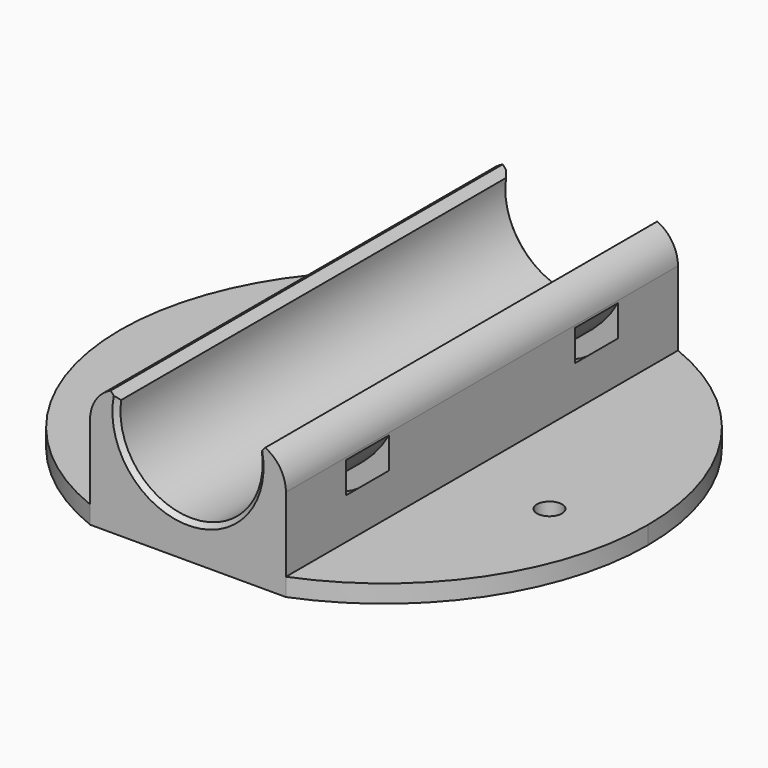
from build123d import *

# Parameters (mm, degrees)
F0_W          = 21.9
F0_H          = 54.784943187
F2_DEPTH      = 13.95
F0_R          = 1.4
F3_DEPTH      = 2
F1_R          = 7.95
F4_DEPTH      = 27.3934715935
F4_DEPTH_BACK = 27.3934715935
F7_R          = 14.5
F7_R_2        = 12.5
F8_R          = 14.5
F8_R_2        = 12.5
F9_DEPTH      = 3
F10_T1_DEPTH  = 59.6298977105
F11_T1_DEPTH  = 72.9200798033
F12_SIZE      = 0.5


# Not quite as in the source:
# - a fillet or chamfer that OpenCascade refuses, or shapes differently, is made with other operations: its cross-section is extruded or revolved along the edge and cut away or added


with BuildPart() as f2:
    # F0 (on Top) → F2 (new body)
    with BuildSketch(Plane.XY):
        Rectangle(F0_W, F0_H)
    extrude(amount=F2_DEPTH)

    # F0 (on Top) → F3 (join)
    with BuildSketch(Plane.XY):
        with BuildLine():
            ThreePointArc((10.95, -27.3924715935), (24.4261642507, -16.5412363504), (29.5, 0))
            ThreePointArc((29.5, 0), (24.4261642507, 16.5412363504), (10.95, 27.3924715935))
            Line((10.95, 27.3924715935), (10.95, -27.3924715935))
        make_face()
        with Locations((20.9, -3)):
            Circle(F0_R, mode=Mode.SUBTRACT)
        with BuildLine():
            Line((-10.95, -27.3924715935), (-10.95, 27.3924715935))
            ThreePointArc((-10.95, 27.3924715935), (-29.5, 0), (-10.95, -27.3924715935))
        make_face()
        with Locations((-20.9, -3)):
            Circle(F0_R, mode=Mode.SUBTRACT)
    extrude(amount=F3_DEPTH)

    # F1 (on Front) → F4 (cut, two sides)
    with BuildSketch(Plane.XZ) as f4_sk:
        with Locations((0, 11.95)):
            Circle(F1_R)
    extrude(amount=-F4_DEPTH, mode=Mode.SUBTRACT)
    extrude(f4_sk.sketch, amount=F4_DEPTH_BACK, mode=Mode.SUBTRACT)

    # F7 (on offset) + F8 (on offset) → F9 (cut, symmetric)
    with BuildSketch(Plane.XZ.offset(16)):
        with Locations((0, 16.1)):
            Circle(F7_R)
        with Locations((0, 16.1)):
            Circle(F7_R_2, mode=Mode.SUBTRACT)
    with BuildSketch(Plane.XZ.offset(-16)):
        with Locations((0, 16.1)):
            Circle(F8_R)
        with Locations((0, 16.1)):
            Circle(F8_R_2, mode=Mode.SUBTRACT)
    extrude(amount=F9_DEPTH, both=True, mode=Mode.SUBTRACT)

    # F10: chamfer of 1 on 2 edges, made by hand

    # F10_s2 → F10_t1 (cut)
    with BuildSketch(Plane.XZ.offset(-29.8149488552)):
        with BuildLine():
            Line((-7.8447816072, 13.0377503134), (-8.6628360241, 13.9802075969))
            Line((-8.6628360241, 13.9802075969), (-8.6628360241, 14.0002075969))
            ThreePointArc((-8.6628360241, 14.0002075969), (-8.178576054, 13.97), (-7.694316084, 13.97))
            Line((-7.694316084, 13.97), (-7.6749593139, 13.9449685535))
            ThreePointArc((-7.6749593139, 13.9449685535), (-7.7779305741, 13.4955406772), (-7.8249803447, 13.0349378407))
            Line((-7.8249803447, 13.0349378407), (-7.8447816072, 13.0377503134))
        make_face()
        with BuildLine():
            Line((8.6628360241, 13.9802075969), (7.8447816072, 13.0377503134))
            Line((7.8447816072, 13.0377503134), (7.8249803447, 13.0349378407))
            ThreePointArc((7.8249803447, 13.0349378407), (7.7779305741, 13.4955406772), (7.6749593139, 13.9449685535))
            Line((7.6749593139, 13.9449685535), (7.694316084, 13.97))
            ThreePointArc((7.694316084, 13.97), (8.178576054, 13.97), (8.6628360241, 14.0002075969))
            Line((8.6628360241, 14.0002075969), (8.6628360241, 13.9802075969))
        make_face()
    extrude(amount=F10_T1_DEPTH, mode=Mode.SUBTRACT)

    # F11: fillet of radius 4 on 2 edges, made by hand

    # F11_s2 → F11_t1 (cut)
    with BuildSketch(Plane.XZ.offset(-36.4600399016)):
        with BuildLine():
            ThreePointArc((10.95, 10.3229726767), (10.3224222102, 12.4739651072), (8.6366157821, 13.95))
            Line((8.6366157821, 13.95), (10.95, 13.95))
            Line((10.95, 13.95), (10.95, 10.3229726767))
        make_face()
        with BuildLine():
            ThreePointArc((-10.95, 10.3229726767), (-10.3224222102, 12.4739651072), (-8.6366157821, 13.95))
            Line((-8.6366157821, 13.95), (-10.95, 13.95))
            Line((-10.95, 13.95), (-10.95, 10.3229726767))
        make_face()
    extrude(amount=F11_T1_DEPTH, mode=Mode.SUBTRACT)

    # F12
    f12_edges = [f2.edges().sort_by_distance(p)[0] for p in [
        (0, 27.392472, 4),
        (0, -27.392472, 4),
    ]]
    chamfer(f12_edges, length=F12_SIZE)


solid = f2.part
